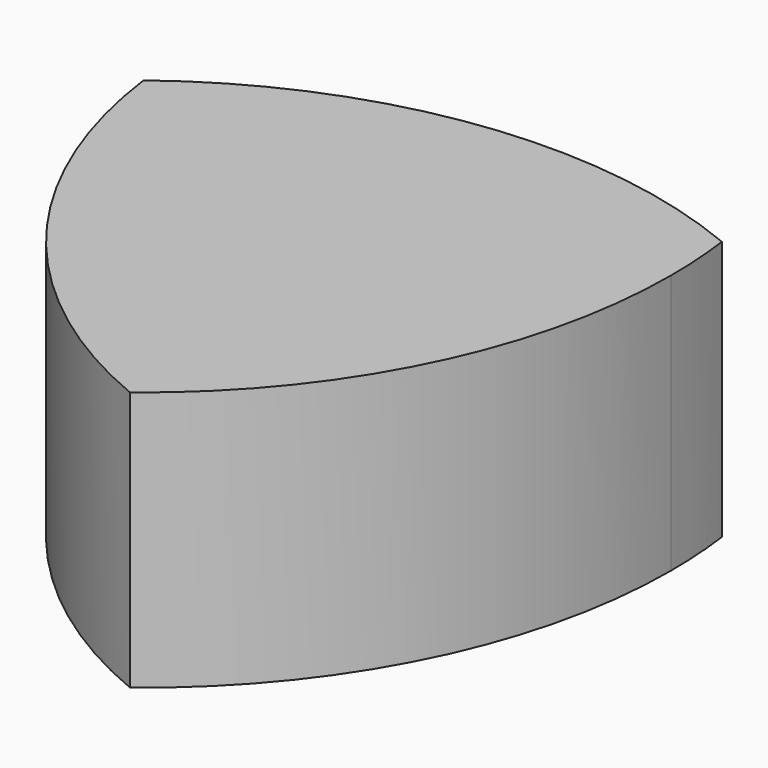
from build123d import *

# Parameters (mm, degrees)
F1_DEPTH = 25.4


with BuildPart() as f1:
    # F0 (on Top) → F1 (new body)
    with BuildSketch(Plane.XY):
        with BuildLine():
            ThreePointArc((0, 0), (-26.4709308966, 3.4779775248), (-51.1344182774, -6.7454710333))
            ThreePointArc((-51.1344182774, -6.7454710333), (-40.9109697193, -31.408958414), (-19.7254598634, -47.6564407526))
            ThreePointArc((-19.7254598634, -47.6564407526), (-4.8730785393, -29.5515789359), (0.4430003477, -6.7454710333))
            ThreePointArc((0.4430003477, -6.7454710333), (0.3321311002, -3.3654699693), (0, 0))
        make_face()
    extrude(amount=F1_DEPTH)


solid = f1.part
